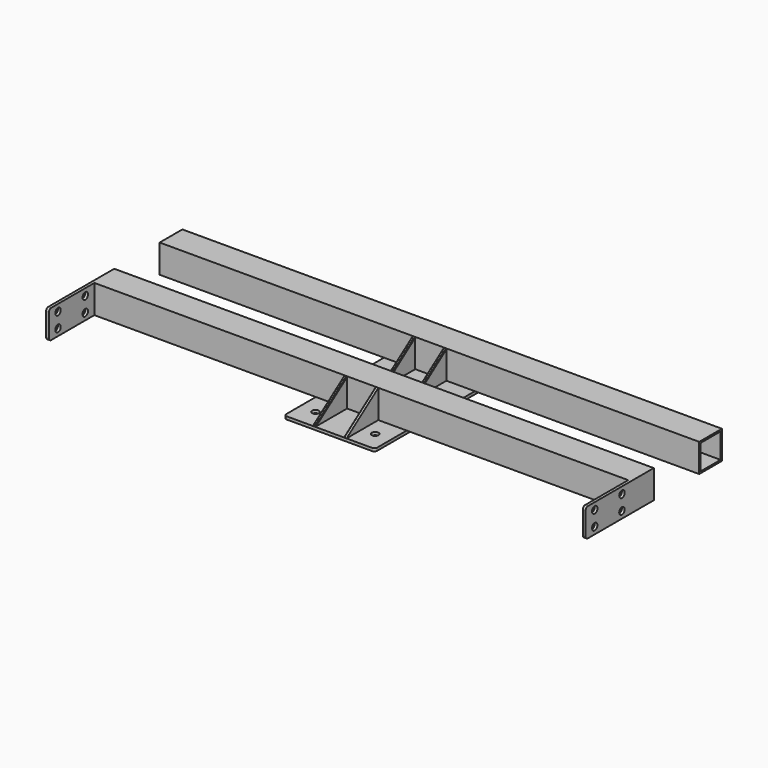
from build123d import *

# Parameters (mm, degrees)
F0_W      = 50
F0_H      = 50
F0_W_2    = 44
F0_H_2    = 44
F1_DEPTH  = 940
F2_W      = 150
F2_H      = 50
F2_R      = 6
F3_DEPTH  = 5
F6_R      = 5
F7_R      = 6
F8_DEPTH  = 5
F9_W      = 5
F9_H      = 70
F10_DEPTH = 50
F12_DEPTH = 110
F13_SIZE  = 1
F15_W     = 50
F15_H     = 50
F15_W_2   = 44
F15_H_2   = 44
F16_DEPTH = 950
F17_W     = 160
F17_H     = 5
F18_DEPTH = 120
F19_R     = 6
F20_DEPTH = 25
F21_W     = 5
F21_H     = 50
F22_DEPTH = 70
F24_DEPTH = 60
F25_R     = 5
F26_SIZE  = 1


with BuildPart() as f1:
    # F0 (on Right) → F1 (new body)
    with BuildSketch(Plane.YZ):
        Rectangle(F0_W, F0_H)
        Rectangle(F0_W_2, F0_H_2, mode=Mode.SUBTRACT)
    extrude(amount=F1_DEPTH)

    # F2 (on face) → F3 (join)
    with BuildSketch(Plane(origin=(0, 0, 0), x_dir=(0, -1, 0), z_dir=(-1, 0, 0))):
        with Locations((50, 0)):
            Rectangle(F2_W, F2_H)
        with Locations((45, -13)):
            Circle(F2_R, mode=Mode.SUBTRACT)
        with Locations((105, -13)):
            Circle(F2_R, mode=Mode.SUBTRACT)
        with Locations((45, 13)):
            Circle(F2_R, mode=Mode.SUBTRACT)
        with Locations((105, 13)):
            Circle(F2_R, mode=Mode.SUBTRACT)
    extrude(amount=F3_DEPTH)

    # F5: F1 across plane


with BuildPart() as f1_1:
    add(f1.part)
    add(f1.part.mirror(Plane.YZ.offset(470)))

    # F6
    f6_edges = [f1_1.edges().sort_by_distance(p)[0] for p in [
        (-2.5, -125, 25),
        (-2.5, -125, -25),
        (942.5, -125, 25),
        (942.5, -125, -25),
    ]]
    fillet(f6_edges, radius=F6_R)

    # F7 (on face) → F8 (join)
    with BuildSketch(Plane(origin=(0, 0, -25), x_dir=(1, 0, 0), z_dir=(0, 0, -1))):
        with BuildLine():
            Line((390, 90), (390, -25))
            Line((390, -25), (550, -25))
            Line((550, -25), (550, 90))
            ThreePointArc((550, 90), (548.5355339059, 93.5355339059), (545, 95))
            Line((545, 95), (395, 95))
            ThreePointArc((395, 95), (391.4644660941, 93.5355339059), (390, 90))
        make_face()
        with Locations((417.5, 60)):
            Circle(F7_R, mode=Mode.SUBTRACT)
        with Locations((522.5, 60)):
            Circle(F7_R, mode=Mode.SUBTRACT)
    extrude(amount=F8_DEPTH)

    # F9 (on face) → F10 (join)
    with BuildSketch(Plane.XY.offset(-25)):
        with Locations((442.5, -60)):
            Rectangle(F9_W, F9_H)
        with Locations((497.5, -60)):
            Rectangle(F9_W, F9_H)
    extrude(amount=F10_DEPTH)

    # F11 (on face) → F12 (cut)
    with BuildSketch(Plane(origin=(440, 0, 0), x_dir=(0, -1, 0), z_dir=(-1, 0, 0))):
        Polygon((95, -25), (95, 25), (25, 25), align=None)
    extrude(amount=-F12_DEPTH, mode=Mode.SUBTRACT)

    # F13
    f13_edges = [f1_1.edges().sort_by_distance(p)[0] for p in [
        (440, -60, 0),
        (445, -60, 0),
        (495, -60, 0),
    ]]
    chamfer(f13_edges, length=F13_SIZE)


with BuildPart() as f16:
    # F15 (on offset) → F16 (new body)
    with BuildSketch(Plane.YZ.offset(-5)):
        with Locations((150, 0)):
            Rectangle(F15_W, F15_H)
        with Locations((150, 0)):
            Rectangle(F15_W_2, F15_H_2, mode=Mode.SUBTRACT)
    extrude(amount=F16_DEPTH)

    # F17 (on face) → F18 (join)
    with BuildSketch(Plane(origin=(0, 175, 0), x_dir=(-1, 0, 0), z_dir=(0, 1, 0))):
        with Locations((-470, -27.5)):
            Rectangle(F17_W, F17_H)
    extrude(amount=-F18_DEPTH)

    # F19 (on face) → F20 (cut)
    with BuildSketch(Plane.XY.offset(-25)):
        with Locations((417.5, 90)):
            Circle(F19_R)
        with Locations((522.5, 90)):
            Circle(F19_R)
    extrude(amount=-F20_DEPTH, mode=Mode.SUBTRACT)

    # F21 (on face) → F22 (join)
    with BuildSketch(Plane.XZ.offset(-125)):
        with Locations((442.5, 0)):
            Rectangle(F21_W, F21_H)
        with Locations((497.5, 0)):
            Rectangle(F21_W, F21_H)
    extrude(amount=F22_DEPTH)

    # F23 (on face) → F24 (cut)
    with BuildSketch(Plane(origin=(440, 0, 0), x_dir=(0, -1, 0), z_dir=(-1, 0, 0))):
        Polygon((-55, -25), (-55, 25), (-125, 25), align=None)
    extrude(amount=-F24_DEPTH, mode=Mode.SUBTRACT)

    # F25
    f25_edges = [f16.edges().sort_by_distance(p)[0] for p in [
        (390, 55, -27.5),
        (550, 55, -27.5),
    ]]
    fillet(f25_edges, radius=F25_R)

    # F26
    f26_edges = [f16.edges().sort_by_distance(p)[0] for p in [
        (445, 90, 0),
        (440, 90, 0),
        (500, 90, 0),
        (495, 90, 0),
    ]]
    chamfer(f26_edges, length=F26_SIZE)


solid = Compound([f1_1.part, f16.part])
